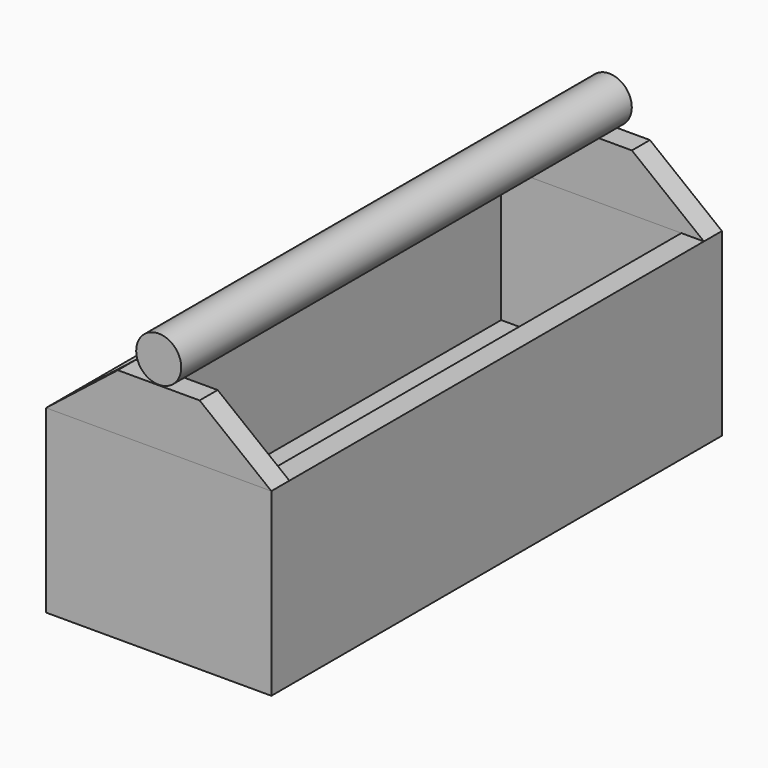
from build123d import *

# Parameters (mm, degrees)
F0_W      = 25.4
F0_H      = 63.5
F1_DEPTH  = 20.32
F2_W      = 20.32
F2_H      = 58.42
F3_DEPTH  = 15.24
F4_W      = 63.5
F4_H      = 2.54
F7_DEPTH  = 2.54
F9_DEPTH  = 2.54
F11_DEPTH = 2.54
F13_DEPTH = 2.54


with BuildPart() as f1:
    # F0 (on Top) → F1 (new body)
    with BuildSketch(Plane.XY):
        Rectangle(F0_W, F0_H)
    extrude(amount=F1_DEPTH)

    # F2 (on face) → F3 (cut)
    with BuildSketch(Plane.XY.offset(20.32)):
        Rectangle(F2_W, F2_H)
    extrude(amount=-F3_DEPTH, mode=Mode.SUBTRACT)


with BuildPart() as f5:
    # F4 (on Right) → F5 (revolve)
    with BuildSketch(Plane.YZ):
        with Locations((0, 30.5581537774)):
            Rectangle(F4_W, F4_H)
    revolve(axis=Axis((0, 0, 29.2881537774), (0, 1, 0)))


with BuildPart() as f7:
    # F6 (on face) → F7 (new body)
    with BuildSketch(Plane.XZ.offset(31.75)):
        Polygon((0, 30.3222630173), (-12.7, 20.32), (12.7, 20.32), align=None)
    extrude(amount=-F7_DEPTH)

    # F10 (on face) → F11 (cut)
    with BuildSketch(Plane.XZ.offset(31.75)):
        Polygon((-4.6117142786, 26.6901701689), (0, 26.6901701689), (4.6117142786, 26.6901701689), (0, 30.3222630173), align=None)
    extrude(amount=-F11_DEPTH, mode=Mode.SUBTRACT)


with BuildPart() as f9:
    # F8 (on face) → F9 (new body)
    with BuildSketch(Plane(origin=(0, 31.75, 0), x_dir=(-1, 0, 0), z_dir=(0, 1, 0))):
        Polygon((0, 30.3222630173), (-12.7, 20.32), (12.7, 20.32), align=None)
    extrude(amount=-F9_DEPTH)

    # F12 (on face) → F13 (cut)
    with BuildSketch(Plane(origin=(0, 31.75, 0), x_dir=(-1, 0, 0), z_dir=(0, 1, 0))):
        Polygon((-4.5833718294, 26.7124921083), (0, 26.7124921083), (4.5833718294, 26.7124921083), (0, 30.3222630173), align=None)
    extrude(amount=-F13_DEPTH, mode=Mode.SUBTRACT)


solid = Compound([f1.part, f5.part, f7.part, f9.part])
